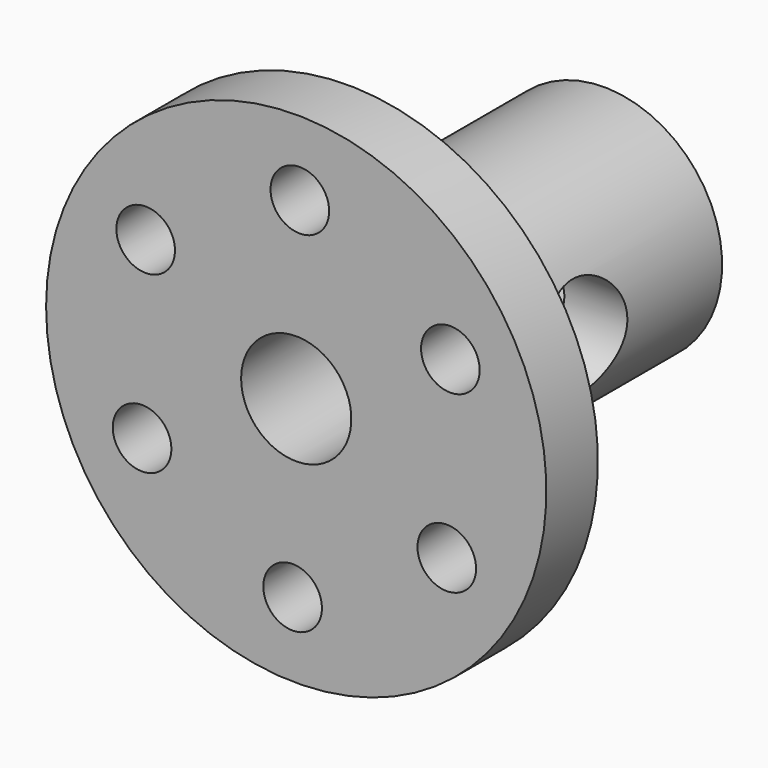
from build123d import *

# Parameters (mm, degrees)
F2_R            = 9.5778194828
F3_DEPTH        = 25.4
F3_COPIES_COUNT = 6
F4_R            = 5.08
F5_R            = 17.307456635
F6_DEPTH        = 70.104


# Not quite as in the source:
# - a pattern or mirror of a feature is missing from the dataset's text; its kind, count and spacing are read off the source's solid


with BuildPart() as f1:
    # F0 (on Top) → F1 (revolve)
    with BuildSketch(Plane.XY):
        Polygon((-35.2849960327, 56.0149177909), (-55.8679103851, 56.0149177909), (-55.8679103851, -48.6638955772), (-99.0202575922, -48.6638955772), (-99.0202575922, -69.7239711881), (-35.2849960327, -69.7239711881), (-35.2849960327, -48.6638955772), align=None)
    revolve(axis=Axis((-17.2766894102, -6.7990683019, 0), (0, -1, 0)))

    # F2 (on face) → F3 (cut)
    with BuildSketch(Plane(origin=(0, -48.6638955772, 0), x_dir=(-1, 0, 0), z_dir=(0, 1, 0))):
        with Locations((18.4528566897, -57.4851334095)):
            Circle(F2_R)
    f3 = extrude(amount=-F3_DEPTH, mode=Mode.SUBTRACT)

    # F3_copies: F3 ×6 about axis
    f3_copies_axis = Axis((-17.276689, 0, 0), (0, 1, 0))
    for i in range(1, F3_COPIES_COUNT):
        add(f3.rotate(f3_copies_axis, i * 360 / F3_COPIES_COUNT), mode=Mode.SUBTRACT)

    # F4
    f4_edges = [f1.edges().sort_by_distance(p)[0] for p in [
        (21.314532, -48.663896, 0),
    ]]
    fillet(f4_edges, radius=F4_R)

    # F5 (on Right) → F6 (cut, symmetric)
    with BuildSketch(Plane.YZ):
        Circle(F5_R)
    extrude(amount=F6_DEPTH, both=True, mode=Mode.SUBTRACT)


solid = f1.part
